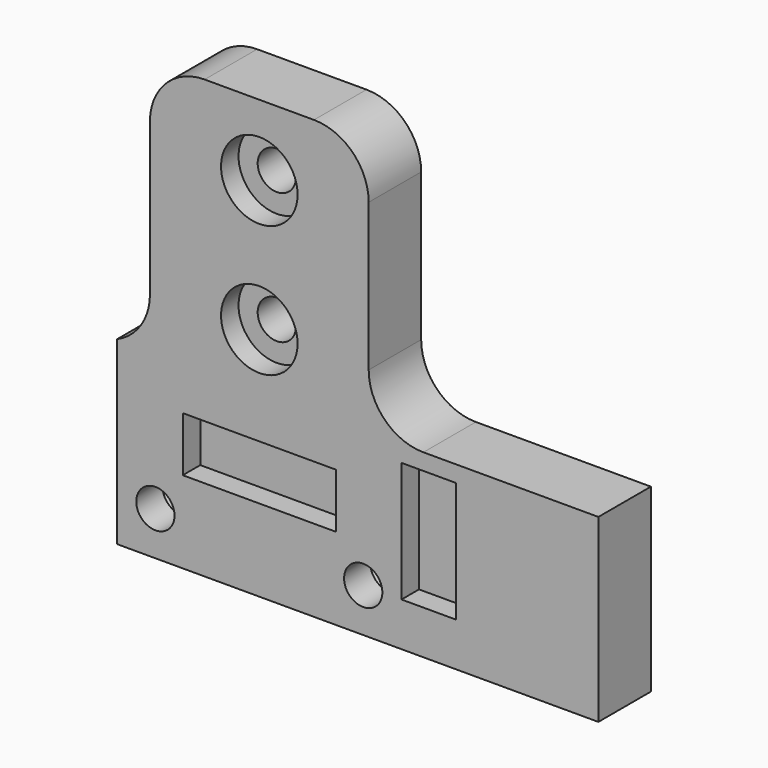
from build123d import *

# Parameters (mm, degrees)
F0_R        = 1.75
F0_W        = 14
F0_H        = 5
F0_W_2      = 5
F0_H_2      = 11
F0_R_2      = 3.5
F1_DEPTH    = 6
F2_DEPTH    = 2
F4_DEPTH    = 3
F5_T1_DEPTH = 6
F5_T3_DEPTH = 6
F5_T5_DEPTH = 31
F5_T7_DEPTH = 31


# Not quite as in the source:
# - a fillet or chamfer that OpenCascade refuses, or shapes differently, is made with other operations: its cross-section is extruded or revolved along the edge and cut away or added


with BuildPart() as f1:
    # F0 (on Front) → F1 (new body)
    with BuildSketch(Plane.XZ):
        Polygon((-11.5, -20), (32.5, -20), (32.5, -3.5), (11.5, -3.5), (11.5, 20), (-8.5, 20), (-8.5, -3.5), (-11.5, -3.5), align=None)
        with Locations((-8, -16)):
            Circle(F0_R, mode=Mode.SUBTRACT)
        with Locations((1.5, -10)):
            Rectangle(F0_W, F0_H, mode=Mode.SUBTRACT)
        with Locations((11, -16)):
            Circle(F0_R, mode=Mode.SUBTRACT)
        with Locations((17, -10.5)):
            Rectangle(F0_W_2, F0_H_2, mode=Mode.SUBTRACT)
        with Locations((1.5, 1.5)):
            Circle(F0_R_2, mode=Mode.SUBTRACT)
        with Locations((1.5, 13.5)):
            Circle(F0_R_2, mode=Mode.SUBTRACT)
        with Locations((1.5, -10)):
            Rectangle(F0_W, F0_H)
        with Locations((17, -10.5)):
            Rectangle(F0_W_2, F0_H_2)
        with Locations((1.5, 1.5)):
            Circle(F0_R_2)
        with Locations((1.5, 1.5)):
            Circle(F0_R, mode=Mode.SUBTRACT)
        with Locations((1.5, 13.5)):
            Circle(F0_R_2)
        with Locations((1.5, 13.5)):
            Circle(F0_R, mode=Mode.SUBTRACT)
    extrude(amount=-F1_DEPTH)

    # F0 (on Front) → F2 (cut)
    with BuildSketch(Plane.XZ):
        with Locations((17, -10.5)):
            Rectangle(F0_W_2, F0_H_2)
        with Locations((1.5, -10)):
            Rectangle(F0_W, F0_H)
        with Locations((1.5, 13.5)):
            Circle(F0_R_2)
        with Locations((1.5, 13.5)):
            Circle(F0_R, mode=Mode.SUBTRACT)
        with Locations((1.5, 1.5)):
            Circle(F0_R_2)
        with Locations((1.5, 1.5)):
            Circle(F0_R, mode=Mode.SUBTRACT)
    extrude(amount=-F2_DEPTH, mode=Mode.SUBTRACT)

    # F3 (on face) → F4 (cut)
    with BuildSketch(Plane(origin=(0, 6, 0), x_dir=(-1, 0, 0), z_dir=(0, 1, 0))):
        Polygon((-11, -12.5358983849), (-14, -14.2679491924), (-14, -17.7320508076), (-11, -19.4641016151), (-8, -17.7320508076), (-8, -14.2679491924), align=None)
        Polygon((5, -14.2679491924), (5, -17.7320508076), (8, -19.4641016151), (11, -17.7320508076), (11, -14.2679491924), (8, -12.5358983849), align=None)
    extrude(amount=-F4_DEPTH, mode=Mode.SUBTRACT)

    # F5: fillet of radius 5 on 4 edges, made by hand

    # F5_s2 → F5_t1 (join)
    with BuildSketch(Plane.XZ.offset(-6)):
        with BuildLine():
            ThreePointArc((-11.5, -3.5), (-9.3166998673, -1.6560370926), (-8.5, 1.082575695))
            Line((-8.5, 1.082575695), (-8.5, -3.5))
            Line((-8.5, -3.5), (-11.5, -3.5))
        make_face()
    extrude(amount=F5_T1_DEPTH)

    # F5_s4 → F5_t3 (join)
    with BuildSketch(Plane.XZ.offset(-6)):
        with BuildLine():
            ThreePointArc((16.5, -3.5), (12.9644660941, -2.0355339059), (11.5, 1.5))
            Line((11.5, 1.5), (11.5, -3.5))
            Line((11.5, -3.5), (16.5, -3.5))
        make_face()
    extrude(amount=F5_T3_DEPTH)

    # F5_s6 → F5_t5 (cut)
    with BuildSketch(Plane.XZ.offset(-18.5)):
        with BuildLine():
            ThreePointArc((-3.5, 20), (-7.0355339059, 18.5355339059), (-8.5, 15))
            Line((-8.5, 15), (-8.5, 20))
            Line((-8.5, 20), (-3.5, 20))
        make_face()
    extrude(amount=F5_T5_DEPTH, mode=Mode.SUBTRACT)

    # F5_s8 → F5_t7 (cut)
    with BuildSketch(Plane.XZ.offset(-18.5)):
        with BuildLine():
            ThreePointArc((6.5, 20), (10.0355339059, 18.5355339059), (11.5, 15))
            Line((11.5, 15), (11.5, 20))
            Line((11.5, 20), (6.5, 20))
        make_face()
    extrude(amount=F5_T7_DEPTH, mode=Mode.SUBTRACT)


solid = f1.part
